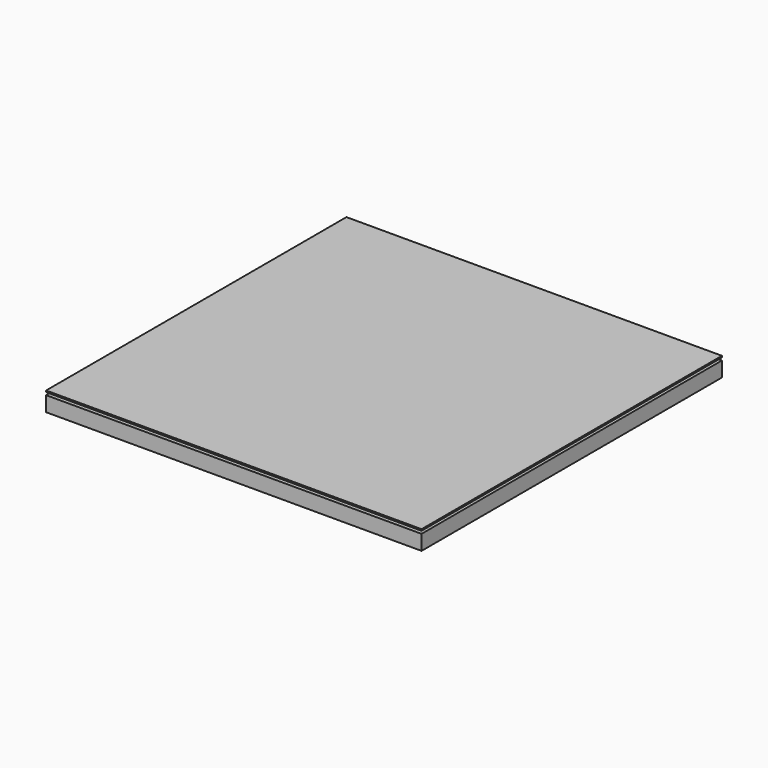
from build123d import *

# Parameters (mm, degrees)
F0_W     = 500
F0_H     = 20
F1_DEPTH = 250
F6_W     = 500
F6_H     = 2
F7_DEPTH = 250


# Not quite as in the source:
# - the program builds the solid bodies; features that only make, move or delete a surface that nothing else refers to are left out


with BuildPart() as f1:
    # F0 (on Front) → F1 (new body, symmetric)
    with BuildSketch(Plane.XZ):
        with Locations((250, 10)):
            Rectangle(F0_W, F0_H)
    extrude(amount=F1_DEPTH, both=True)


with BuildPart() as f7:
    # F6 (on Front) → F7 (new body, symmetric)
    with BuildSketch(Plane.XZ):
        with Locations((250, 24.5)):
            Rectangle(F6_W, F6_H)
    extrude(amount=F7_DEPTH, both=True)


solid = Compound([f1.part, f7.part])
